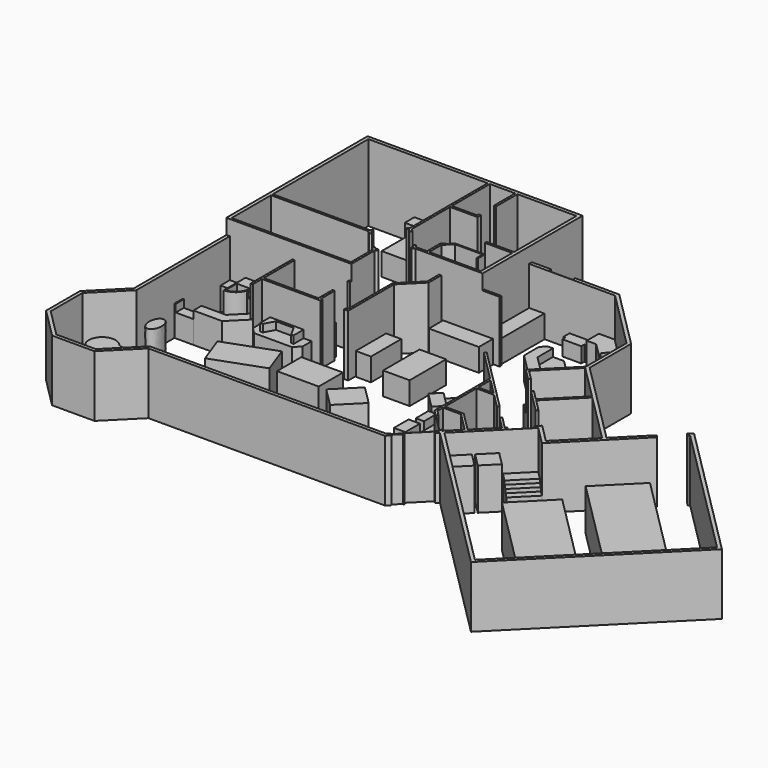
from build123d import *

# Parameters (mm, degrees)
F1_DEPTH  = 3076.575
F0_W      = 609.6
F0_H      = 1219.2
F2_DEPTH  = 914.4
F0_W_2    = 558.8
F0_H_2    = 482.6
F0_W_3    = 1676.4
F0_H_3    = 2438.4
F0_W_4    = 482.6
F0_H_4    = 1473.2
F0_W_5    = 355.6
F0_H_5    = 762
F0_W_6    = 457.2
F0_H_6    = 457.2
F3_DEPTH  = 609.6
F4_W      = 88.9
F4_H      = 76.2
F4_H_2    = 88.9
F5_DEPTH  = 2466.975
F6_DEPTH  = 1219.2
F4_W_2    = 1676.4
F4_H_3    = 1219.2
F4_W_3    = 889
F4_H_4    = 762
F4_W_4    = 1016
F4_H_5    = 381
F4_W_5    = 330.2
F4_H_6    = 635
F4_W_6    = 457.2
F4_H_7    = 736.6
F4_H_8    = 508
F4_W_7    = 1524
F4_H_9    = 457.2
F4_W_8    = 50.8
F4_H_10   = 406.4
F7_DEPTH  = 914.4
F4_W_9    = 622.3
F4_H_11   = 469.9
F4_W_10   = 711.2
F8_W      = 685.8
F8_H      = 88.9
F8_W_2    = 76.2
F8_W_3    = 965.2
F8_H_2    = 6.35
F9_DEPTH  = 2466.975
F8_W_4    = 609.6
F8_H_3    = 1524
F10_DEPTH = 914.4
F8_W_5    = 1066.8
F8_H_4    = 1828.8
F8_W_6    = 2006.6
F8_H_5    = 711.2
F8_R      = 114.3
F11_DEPTH = 609.6
F13_DEPTH = 2466.975
F14_DEPTH = 914.4
F12_W     = 685.8
F12_H     = 355.6
F15_DEPTH = 762
F16_DEPTH = 609.6
F18_DEPTH = 2466.975
F19_DEPTH = 1676.4


# Not quite as in the source:
# - a feature names something its author has since deleted; it is built from what else it names


with BuildPart() as f1:
    # F0 (on Top) → F1 (new body)
    with BuildSketch(Plane.XY):
        Polygon((-1281.9462310372, 633.3950885865), (-1281.9462310372, 1090.5950885865), (-824.7462310372, 1090.5950885865), (94.7987193947, 1090.5950885865), (1090.5950885865, 1090.5950885865), (1090.5950885865, 94.7987193947), (1090.5950885865, -824.7462310372), (1090.5950885865, -2043.9462310372), (480.9950885865, -2043.9462310372), (-14.3049114135, -2043.9462310372), (-14.3049114135, -2132.8462310372), (1090.5950885865, -2132.8462310372), (1090.5950885865, -3707.6462310372), (-986.9836923831, -3707.6462310372), (-986.9836923831, -3098.0462310372), (-682.1836923831, -2793.2462310372), (430.1950885865, -2793.2462310372), (430.1950885865, -3098.0462310372), (480.9950885865, -3098.0462310372), (480.9950885865, -2742.4462310372), (-703.2257413517, -2742.4462310372), (-915.1416434146, -2954.3621331001), (-942.0824117778, -2927.4213647369), (-1075.8836923831, -3061.2226453422), (-1075.8836923831, -3707.6462310372), (-1506.7811311724, -3707.6462310372), (-1614.5442046253, -3599.8831575844), (-1677.4059974727, -3662.7449504319), (-1569.6429240199, -3770.5080238847), (-1623.5244607463, -3824.3895606111), (-1560.6626678988, -3887.2513534586), (-1469.9575454775, -3796.5462310372), (1230.2950885865, -3796.5462310372), (1230.2950885865, 152.6643540582), (1230.2950885865, 1230.2950885865), (152.6643540582, 1230.2950885865), (-6336.0568161326, 1230.2950885865), (-7413.6875506609, 1230.2950885865), (-7413.6875506609, 152.6643540582), (-7413.6875506609, -5866.6462310372), (-2386.8462310372, -5866.6462310372), (-2386.8462310372, -4713.4349165969), (-2296.1411086158, -4622.7297941756), (-2359.0029014633, -4559.8680013281), (-2412.8844381897, -4613.7495380545), (-2520.6475116425, -4505.9864646017), (-2583.50930449, -4568.8482574492), (-2475.7462310372, -4676.611330902), (-2475.7462310372, -5777.7462310372), (-7273.9875506609, -5777.7462310372), (-7273.9875506609, -3796.5462310372), (-3355.811330902, -3796.5462310372), (-3248.0482574491, -3904.30930449), (-3185.1864646017, -3841.4475116425), (-3292.9495380545, -3733.6844381897), (-3239.0680013281, -3679.8029014633), (-3301.9297941756, -3616.9411086158), (-3392.6349165969, -3707.6462310372), (-6918.3875506609, -3707.6462310372), (-7273.9875506609, -3707.6462310372), (-7273.9875506609, -2945.6462310372), (-7273.9875506609, -2640.8462310372), (-7273.9875506609, -1167.6462310372), (-7273.9875506609, 94.7987193946), (-7273.9875506609, 1090.5950885865), (-6278.1911814691, 1090.5950885865), (-5422.1462310372, 1090.5950885865), (-4863.3462310372, 1090.5950885865), (-4787.1462310372, 1090.5950885865), (-3110.7462310372, 1090.5950885865), (-3034.5462310372, 1090.5950885865), (-2475.7462310372, 1090.5950885865), (-2475.7462310372, 607.9950885865), (-2475.7462310372, -2790.7575454775), (-2566.4513534586, -2881.4626678988), (-2503.5895606111, -2944.3244607463), (-2449.7080238847, -2890.4429240199), (-2341.9449504319, -2998.2059974727), (-2279.0831575844, -2935.3442046253), (-2386.8462310372, -2827.5811311724), (-2386.8462310372, -2585.9072780781), (-2386.8462310372, -909.5072780781), (-1777.2462310372, -909.5072780781), (-1281.9462310372, -909.5072780781), (-1281.9462310372, -820.6072780781), (-1281.9462310372, -744.4072780781), (-1370.8462310372, -744.4072780781), (-1370.8462310372, -820.6072780781), (-2386.8462310372, -820.6072780781), (-2386.8462310372, 1090.5950885865), (-1370.8462310372, 1090.5950885865), (-1370.8462310372, 17.5927219219), (-1281.9462310372, 17.5927219219), align=None)
    extrude(amount=F1_DEPTH)

    # F4 (on Top) → F5 (join)
    with BuildSketch(Plane.XY):
        Polygon((-7273.9875506609, -5866.6462310372), (-7413.6875506609, -5866.6462310372), (-7413.6875506609, -10507.7805963737), (-8618.8845674344, -11712.9776131472), (-8618.8845674344, -13417.3835796), (-7413.6875506609, -14622.5805963736), (-5709.281584208, -14622.5805963736), (-4504.0845674344, -13417.3835796), (5003.0722012166, -13417.3835796), (5151.7524573376, -13268.703323479), (5120.3215609139, -13237.2724270553), (5371.7687323038, -12985.8252556653), (5403.1996287275, -13017.2561520891), (5439.1206532118, -12981.3351276048), (5358.2983481222, -12900.5128225152), (6040.7978133234, -12218.0133573139), (6121.6201184131, -12298.8356624035), (6858.0011203407, -11562.4546604759), (5991.0966946136, -10695.5502347487), (5229.0966946136, -10695.5502347487), (5229.0966946136, -8271.0625060034), (3959.293014693, -7001.2588260828), (3896.4312218455, -7064.1206189303), (5140.1966946136, -8307.8860916984), (5140.1966946136, -11101.8860916984), (6130.6003745341, -12092.2897716189), (6022.8373010813, -12200.0528450718), (6036.3076852629, -12213.5232292534), (5353.8082200616, -12896.0226944546), (5340.33783588, -12882.552310273), (5304.4168113958, -12918.4733347573), (5335.8477078195, -12949.9042311811), (5084.4005364296, -13201.351402571), (5052.9696400058, -13169.9205061472), (4945.206566553, -13277.6835796001), (-4561.950202098, -13277.6835796), (-5767.1472188716, -14482.8805963736), (-7355.8219159973, -14482.8805963736), (-8479.1845674344, -13359.5179449365), (-8479.1845674344, -11770.8432478107), (-7273.9875506609, -10565.6462310372), (-7273.9875506609, -8648.3200841315), (-7273.9875506609, -8241.9200841315), (-7273.9875506609, -6336.5462310372), align=None)
        Polygon((6696.3565101615, -11526.5336359916), (6193.4621673816, -12029.4279787715), (6139.5806306552, -11975.5464420451), (6081.2089658682, -12033.918106832), (5398.709500667, -11351.4186416307), (5457.0811654539, -11293.0469768438), (5229.0966946136, -11065.0625060034), (5229.0966946136, -10784.4502347487), (5954.2731089186, -10784.4502347487), align=None, mode=Mode.SUBTRACT)
        Polygon((-4759.3875506609, -6901.5734475404), (-4759.3875506609, -7476.3098392888), (-4759.3875506609, -7873.2462310372), (-4670.4875506609, -7873.2462310372), (-4670.4875506609, -7504.9462310372), (-4345.0193547867, -7504.9462310372), (-2998.8193547867, -7504.9462310372), (-2673.3511589125, -7504.9462310372), (-2386.8462310372, -7504.9462310372), (-2386.8462310372, -6704.8462310372), (-2475.7462310372, -6704.8462310372), (-2475.7462310372, -7416.0462310372), (-4670.4875506609, -7416.0462310372), (-4670.4875506609, -5866.6462310372), (-4759.3875506609, -5866.6462310372), (-4759.3875506609, -6336.5462310372), align=None)
        with Locations((-2431.2962310372, -5904.7462310372)):
            Rectangle(F4_W, F4_H)
        with Locations((-4714.9375506609, -7917.6962310372)):
            Rectangle(F4_W, F4_H_2)
    extrude(amount=F5_DEPTH)

    # F8 (on Top) → F9 (join)
    with BuildSketch(Plane.XY):
        with Locations((1573.1950885865, -3752.0962310372)):
            Rectangle(F8_W, F8_H)
        Polygon((2004.9950885865, -1321.5416434146), (1230.2950885865, -1321.5416434146), (1230.2950885865, -1461.2416434146), (2004.9950885865, -1461.2416434146), (2004.9950885865, -1454.8916434146), align=None)
        Polygon((2970.1950885865, -1321.5416434146), (2970.1950885865, -1454.8916434146), (2970.1950885865, -1461.2416434146), (4683.6642412751, -1461.2416434146), (6987.9344635613, -3765.5118657007), (6987.9344635613, -5805.0420654303), (5647.8073852128, -7145.1691437788), (5710.6691780603, -7208.0309366262), (7127.6344635613, -5791.0656511253), (7127.6344635613, -3707.6462310372), (4741.5298759387, -1321.5416434146), align=None)
        Polygon((-1370.8462310372, -7416.0462310372), (-1370.8462310372, -7504.9462310372), (-1205.7462310372, -7504.9462310372), (-1205.7462310372, -5202.6625551158), (-431.6390822039, -4428.5554062825), (-431.6390822039, -3796.5462310372), (-520.5390822039, -3796.5462310372), (-520.5390822039, -4391.7318205875), (-1294.6462310372, -5165.8389694208), (-1294.6462310372, -7416.0462310372), align=None)
        with Locations((-2348.7462310372, -7460.4962310372)):
            Rectangle(F8_W_2, F8_H)
        with Locations((2487.5950885865, -1458.0666434146)):
            Rectangle(F8_W_3, F8_H_2)
    extrude(amount=F9_DEPTH)

    # F12 (on Top) → F13 (join)
    with BuildSketch(Plane.XY):
        Polygon((7028.8516462295, -5889.848468457), (8396.7700366499, -7257.7668588774), (7141.4493613282, -8513.0875341992), (6798.7398987186, -8170.3780715896), (6744.8583619922, -8116.4965348632), (6681.9965691447, -8179.3583277107), (7626.3831918659, -9123.7449504319), (7689.2449847134, -9060.8831575844), (7635.363447987, -9007.001620858), (7204.3111541757, -8575.9493270466), (8459.6318294974, -7320.6286517249), (8890.6841233087, -7751.6809455362), (10417.3276638905, -9278.324486118), (9162.0069885687, -10533.6451614397), (8425.6259866411, -9797.2641595121), (8362.7641937936, -9860.1259523595), (8255.0011203407, -9967.8890258124), (8349.293809612, -10062.1817150836), (7738.6363933793, -10672.8391313163), (7644.343704108, -10578.5464420451), (7590.4621673816, -10632.4279787715), (7105.5283368439, -10147.4941482337), (7042.6665439964, -10210.3559410812), (7527.6003745341, -10695.289771619), (6759.218303009, -11463.6718431441), (6858.0011203407, -11562.4546604759), (7635.363447987, -10785.0923328297), (7689.2449847134, -10731.2107961033), (8425.6259866411, -9994.8297941756), (8757.8954631206, -10327.0992706551), (8959.9512258447, -10529.1550333792), (9162.0069885687, -10731.2107961033), (10614.893298554, -9278.324486118), (7127.6344635613, -5791.0656511253), align=None)
        Polygon((6116.2404335173, -7487.8786063883), (5773.5309709078, -7145.1691437788), (5710.6691780603, -7208.0309366262), (6107.2601773963, -7604.6219359622), (6170.1219702438, -7541.7601431147), align=None)
        Polygon((5229.0966946136, -8271.0625060034), (5229.0966946136, -8396.7860916984), (5851.3966946135, -9019.0860916984), (5229.0966946136, -9019.0860916984), (5229.0966946136, -9107.9860916984), (5940.2966946136, -9107.9860916984), (6503.8511767323, -9671.5405738171), (6566.7129695797, -9608.6787809696), align=None)
    extrude(amount=F13_DEPTH)

    # F17 (on Top) → F18 (join)
    with BuildSketch(Plane.XY):
        Polygon((6328.1660091977, -12092.289771619), (6229.3831918659, -12191.0725889507), (12470.6611960089, -18432.3505930938), (18074.3410155561, -12828.6707735467), (12470.661196009, -7224.9909539995), (12317.9968419508, -7377.6553080577), (12416.7796592826, -7476.4381253894), (12470.661196009, -7422.556588663), (17876.7753808926, -12828.6707735467), (12470.6611960089, -18234.7849584303), align=None)
        Polygon((10516.1104812222, -9179.5416687862), (10614.893298554, -9278.324486118), (11734.2801940813, -8158.9375905907), (11635.4973767496, -8060.1547732589), align=None)
    extrude(amount=F18_DEPTH)


with BuildPart() as f2:
    # F0 (on Top) → F2 (new body)
    with BuildSketch(Plane.XY):
        with Locations((785.7950885865, -1434.3462310372)):
            Rectangle(F0_W, F0_H)
        with BuildLine():
            add(Edge.make_bspline(
                [(734.9950885865, -1180.3462310372), (383.0423644885, -1180.3462310372), (559.0187265375, -1561.3462310372), (734.9950885865, -1942.3462310372), (910.9714506355, -1561.3462310372), (1086.9478126845, -1180.3462310372), (734.9950885865, -1180.3462310372)],
                knots=[0, 0, 0, 2.0943951024, 2.0943951024, 4.1887902048, 4.1887902048, 6.2831853072, 6.2831853072, 6.2831853072], degree=2, weights=[1, 0.5, 1, 0.5, 1, 0.5, 1]))
        make_face(mode=Mode.SUBTRACT)
    extrude(amount=F2_DEPTH)


with BuildPart() as f2b:
    # F0 (on Top) → F2, piece 2 (new body)
    with BuildSketch(Plane.XY):
        Polygon((-1777.2462310372, -2433.5072780781), (-1777.2462310372, -909.5072780781), (-2386.8462310372, -909.5072780781), (-2386.8462310372, -2585.9072780781), (-1929.6462310372, -2585.9072780781), align=None)
        with BuildLine():
            add(Edge.make_bspline(
                [(-2031.2462310372, -1925.5072780781), (-1679.2935069392, -1925.5072780781), (-1855.2698689882, -1544.5072780781), (-2031.2462310372, -1163.5072780781), (-2207.2225930862, -1544.5072780781), (-2383.1989551352, -1925.5072780781), (-2031.2462310372, -1925.5072780781)],
                knots=[0, 0, 0, 2.0943951024, 2.0943951024, 4.1887902048, 4.1887902048, 6.2831853072, 6.2831853072, 6.2831853072], degree=2, weights=[1, 0.5, 1, 0.5, 1, 0.5, 1]))
        make_face(mode=Mode.SUBTRACT)
    extrude(amount=F2_DEPTH)


with BuildPart() as f2c:
    # F0 (on Top) → F2, piece 3 (new body)
    with BuildSketch(Plane.XY):
        with Locations((-5142.7462310372, 849.2950885865)):
            Rectangle(F0_W_2, F0_H_2)
    extrude(amount=F2_DEPTH)


with BuildPart() as f2d:
    # F0 (on Top) → F2, piece 4 (new body)
    with BuildSketch(Plane.XY):
        with Locations((-3948.9462310372, -128.6049114135)):
            Rectangle(F0_W_3, F0_H_3)
    extrude(amount=F2_DEPTH)


with BuildPart() as f2e:
    # F0 (on Top) → F2, piece 5 (new body)
    with BuildSketch(Plane.XY):
        with Locations((-2755.1462310372, 849.2950885865)):
            Rectangle(F0_W_2, F0_H_2)
    extrude(amount=F2_DEPTH)


with BuildPart() as f2f:
    # F0 (on Top) → F2, piece 6 (new body)
    with BuildSketch(Plane.XY):
        with Locations((-7032.6875506609, -1904.2462310372)):
            Rectangle(F0_W_4, F0_H_4)
    extrude(amount=F2_DEPTH)


with BuildPart() as f2g:
    # F0 (on Top) → F2, piece 7 (new body)
    with BuildSketch(Plane.XY):
        with Locations((-7096.1875506609, -3326.6462310372)):
            Rectangle(F0_W_5, F0_H_5)
    extrude(amount=F2_DEPTH)


with BuildPart() as f2h:
    # F0 (on Top) → F2, piece 8 (new body)
    with BuildSketch(Plane.XY):
        with Locations((-1053.3462310372, 861.9950885865)):
            Rectangle(F0_W_6, F0_H_6)
    extrude(amount=F2_DEPTH)


with BuildPart() as f3:
    # F0 (on Top) → F3 (new body)
    with BuildSketch(Plane.XY):
        Polygon((94.7987193947, 1090.5950885865), (-824.7462310372, 1090.5950885865), (-824.7462310372, 633.3950885865), (-824.7462310372, -37.3583565854), (-37.3583565854, -824.7462310372), (480.9950885865, -824.7462310372), (1090.5950885865, -824.7462310372), (1090.5950885865, 94.7987193947), (1090.5950885865, 1090.5950885865), align=None)
        with BuildLine():
            add(Edge.make_bspline(
                [(646.578440717, -646.578440717), (1299.8573551173, 6.7004736833), (3.3502368416, 649.9286775586), (-1293.156881434, 1293.156881434), (-649.9286775586, -3.3502368416), (-6.7004736833, -1299.8573551173), (646.578440717, -646.578440717)],
                knots=[0, 0, 0, 2.0943951024, 2.0943951024, 4.1887902048, 4.1887902048, 6.2831853072, 6.2831853072, 6.2831853072], degree=2, weights=[1, 0.5, 1, 0.5, 1, 0.5, 1]))
        make_face(mode=Mode.SUBTRACT)
    extrude(amount=F3_DEPTH)


with BuildPart() as f6:
    # F4 (on Top) → F6 (new body)
    with BuildSketch(Plane.XY):
        Polygon((-2609.6755261771, -9084.0103363379), (-4614.6037018859, -9813.7445141375), (-4197.6127431432, -10959.4177573997), (-2192.6845674344, -10229.6835796), align=None)
    extrude(amount=F6_DEPTH)


with BuildPart() as f6b:
    # F4 (on Top) → F6, piece 2 (new body)
    with BuildSketch(Plane.XY):
        with Locations((-1049.6845674344, -9620.0835796)):
            Rectangle(F4_W_2, F4_H_3)
    extrude(amount=F6_DEPTH)


with BuildPart() as f6c:
    # F4 (on Top) → F6, piece 3 (new body)
    with BuildSketch(Plane.XY):
        Polygon((1709.761534358, -10121.9205061472), (955.4200201882, -9367.5789919774), (93.3154325656, -10229.6835796), (847.6569467354, -10984.0250937698), align=None)
    extrude(amount=F6_DEPTH)


with BuildPart() as f6d:
    # F4 (on Top) → F6, piece 4 (new body)
    with BuildSketch(Plane.XY):
        with Locations((-4200.5875506609, -7009.6462310372)):
            Rectangle(F4_W_3, F4_H_4)
    extrude(amount=F6_DEPTH)


with BuildPart() as f6e:
    # F4 (on Top) → F6, piece 5 (new body)
    with BuildSketch(Plane.XY):
        Polygon((-2501.1462310372, -6501.6462310372), (-3567.9462310372, -6501.6462310372), (-3567.9462310372, -6527.0462310372), (-3567.9462310372, -7390.6462310372), (-2501.1462310372, -7390.6462310372), (-2501.1462310372, -6527.0462310372), align=None)
        with Locations((-3034.5462310372, -6717.5462310372)):
            Rectangle(F4_W_4, F4_H_5, mode=Mode.SUBTRACT)
    extrude(amount=F6_DEPTH)


with BuildPart() as f6f:
    # F4 (on Top) → F6, piece 6 (new body)
    with BuildSketch(Plane.XY):
        Polygon((3115.8551804438, -8115.5168262267), (2774.6054478431, -8456.7665588273), (3403.223376318, -9085.3844873021), (3744.4731089186, -8744.1347547015), align=None)
    extrude(amount=F6_DEPTH)


with BuildPart() as f6g:
    # F4 (on Top) → F6, piece 7 (new body)
    with BuildSketch(Plane.XY):
        with Locations((3679.6966946136, -9692.1860916984)):
            Rectangle(F4_W_5, F4_H_6)
    extrude(amount=F6_DEPTH)


with BuildPart() as f6h:
    # F4 (on Top) → F6, piece 8 (new body)
    with BuildSketch(Plane.XY):
        with Locations((3616.1966946136, -10581.1860916984)):
            Rectangle(F4_W_6, F4_H_7)
    extrude(amount=F6_DEPTH)


with BuildPart() as f6i:
    # F4 (on Top) → F6, piece 9 (new body)
    with BuildSketch(Plane.XY):
        with Locations((4132.406566553, -12998.2835796)):
            Rectangle(F4_W_4, F4_H_8)
    extrude(amount=F6_DEPTH)


with BuildPart() as f6j:
    # F4 (on Top) → F6, piece 10 (new body)
    with BuildSketch(Plane.XY):
        with BuildLine():
            ThreePointArc((3281.506566553, -13252.2835796), (3472.006566553, -13061.7835796), (3281.506566553, -12871.2835796))
            Line((3281.506566553, -12871.2835796001), (2684.606566553, -12871.2835796001))
            Line((2684.606566553, -12871.2835796), (2684.606566553, -13252.2835796))
            Line((2684.606566553, -13252.2835796), (3281.506566553, -13252.2835796))
        make_face()
    extrude(amount=F6_DEPTH)


with BuildPart() as f6k:
    # F4 (on Top) → F6, piece 11 (new body)
    with BuildSketch(Plane.XY):
        with Locations((-3183.2845674344, -12845.8835796)):
            Rectangle(F4_W_4, F4_H_4)
    extrude(amount=F6_DEPTH)


with BuildPart() as f6l:
    # F4 (on Top) → F6, piece 12 (new body)
    with BuildSketch(Plane.XY):
        Polygon((-6225.7143451483, -13540.5277677636), (-5974.2671737583, -13791.9749391535), (-5435.4518064942, -13253.1595718893), (-5686.8989778841, -13001.7124004994), align=None)
    extrude(amount=F6_DEPTH)


with BuildPart() as f6m:
    # F4 (on Top) → F6, piece 13 (new body)
    with BuildSketch(Plane.XY):
        with BuildLine():
            Line((-7662.5553245194, -12642.5021556566), (-6746.5692001703, -13558.4882800057))
            Line((-6746.5692001703, -13558.4882800057), (-5668.938465642, -12480.8575454774))
            Line((-5668.938465642, -12480.8575454774), (-6099.9907594533, -12049.8052516661))
            ThreePointArc((-6099.9907594532, -12049.805251666), (-6289.8110096941, -11948.216536705), (-6504.1022849014, -11968.9829465764))
            ThreePointArc((-6504.1022849014, -11968.9829465764), (-6718.3935601087, -11989.7493564478), (-6908.2138103495, -11888.1606414868))
            ThreePointArc((-6908.2138103495, -11888.1606414868), (-7662.5553245193, -11888.1606414868), (-7662.5553245194, -12642.5021556566))
        make_face()
    extrude(amount=F6_DEPTH)


with BuildPart() as f6n:
    # F4 (on Top) → F6, piece 14 (new body)
    with BuildSketch(Plane.XY):
        with BuildLine():
            add(Edge.make_bspline(
                [(-6873.1369972229, -10508.4746231079), (-6433.1960921004, -10508.4746231079), (-6653.1665446617, -9898.8746231079), (-6873.1369972229, -9289.2746231079), (-7093.1074497841, -9898.8746231079), (-7313.0779023454, -10508.4746231079), (-6873.1369972229, -10508.4746231079)],
                knots=[0, 0, 0, 2.0943951024, 2.0943951024, 4.1887902048, 4.1887902048, 6.2831853072, 6.2831853072, 6.2831853072], degree=2, weights=[1, 0.5, 1, 0.5, 1, 0.5, 1]))
        make_face()
    extrude(amount=F6_DEPTH)


with BuildPart() as f6o:
    # F4 (on Top) → F6, piece 15 (new body)
    with BuildSketch(Plane.XY):
        with Locations((-1049.6845674344, -12998.2835796)):
            Rectangle(F4_W_7, F4_H_9)
    extrude(amount=F6_DEPTH)


with BuildPart() as f6p:
    # F4 (on Top) → F6, piece 16 (new body)
    with BuildSketch(Plane.XY):
        with BuildLine():
            Line((-5407.0875506609, -5892.0462310372), (-6626.2875506609, -5892.0462310372))
            Line((-6626.2875506609, -5892.0462310372), (-6626.2875506609, -6374.6462310372))
            Line((-6626.2875506609, -6374.6462310372), (-6626.2875506609, -6984.2462310372))
            ThreePointArc((-6626.2875506609, -6984.2462310372), (-6195.2352568496, -6805.6985248485), (-6016.6875506609, -6374.6462310372))
            ThreePointArc((-6016.6875506609, -6374.6462310372), (-5838.1398444722, -6805.6985248485), (-5407.0875506609, -6984.2462310372))
            Line((-5407.0875506609, -6984.2462310372), (-5407.0875506609, -6374.6462310372))
            Line((-5407.0875506609, -6374.6462310372), (-5407.0875506609, -5892.0462310372))
        make_face()
        with BuildLine():
            Line((-6588.1875506609, -6944.8748167815), (-6588.1875506609, -6374.6462310372))
            Line((-6588.1875506609, -6374.6462310372), (-6054.7875506609, -6374.6462310372))
            ThreePointArc((-6054.7875506609, -6374.6462310372), (-6208.9229618419, -6765.0550552203), (-6588.1875506609, -6944.8748167815))
        make_face(mode=Mode.SUBTRACT)
        with BuildLine():
            Line((-5978.5875506609, -6374.6462310372), (-5445.1875506609, -6374.6462310372))
            Line((-5445.1875506609, -6374.6462310372), (-5445.1875506609, -6944.8748167815))
            ThreePointArc((-5445.1875506609, -6944.8748167815), (-5824.4521394798, -6765.0550552203), (-5978.5875506609, -6374.6462310372))
        make_face(mode=Mode.SUBTRACT)
    extrude(amount=F6_DEPTH)


with BuildPart() as f6q:
    # F4 (on Top) → F6, piece 17 (new body)
    with BuildSketch(Plane.XY):
        Polygon((-6461.1875506609, -8241.9200841315), (-6511.9875506609, -8241.9200841315), (-6511.9875506609, -8648.3200841315), (-5356.6614037552, -8648.3200841315), (-5253.752917925, -8545.4115983013), (-4750.8585751452, -8042.5172555215), (-4670.4875506609, -7962.1462310372), (-4759.3875506609, -7962.1462310372), (-4759.3875506609, -7873.2462310372), (-4759.3875506609, -7476.3098392888), (-5524.9977955036, -8241.9200841315), align=None)
    extrude(amount=F6_DEPTH)


with BuildPart() as f6r:
    # F4 (on Top) → F6, piece 18 (new body)
    with BuildSketch(Plane.XY):
        with Locations((-7248.5875506609, -8445.1200841315)):
            Rectangle(F4_W_8, F4_H_10)
    extrude(amount=F6_DEPTH)


with BuildPart() as f6s:
    # F4 (on Top) → F6, piece 19 (new body)
    with BuildSketch(Plane.XY):
        Polygon((-2998.8193547867, -7504.9462310372), (-4345.0193547867, -7504.9462310372), (-4345.0193547867, -8000.2462310372), (-4243.4193547867, -8000.2462310372), (-4027.5193547867, -7606.5462310372), (-3316.3193547867, -7606.5462310372), (-3100.4193547867, -8000.2462310372), (-2998.8193547867, -8000.2462310372), align=None)
    extrude(amount=F6_DEPTH)


with BuildPart() as f7:
    # F4 (on Top) → F7 (new body)
    with BuildSketch(Plane.XY):
        Polygon((5140.1966946136, -8307.8860916984), (3896.4312218455, -7064.1206189303), (2998.4056097386, -7962.1462310372), (3870.1966946136, -8833.9373159122), (3870.1966946136, -11101.8860916984), (5140.1966946136, -11101.8860916984), align=None)
    extrude(amount=F7_DEPTH)


with BuildPart() as f7b:
    # F4 (on Top) → F7, piece 2 (new body)
    with BuildSketch(Plane.XY):
        with Locations((-5070.5375506609, -6101.5962310372)):
            Rectangle(F4_W_9, F4_H_11)
    extrude(amount=F7_DEPTH)


with BuildPart() as f7c:
    # F4 (on Top) → F7, piece 3 (new body)
    with BuildSketch(Plane.XY):
        with Locations((-6962.8375506609, -6101.5962310372)):
            Rectangle(F4_W_9, F4_H_11)
    extrude(amount=F7_DEPTH)


with BuildPart() as f7d:
    # F4 (on Top) → F7, piece 4 (new body)
    with BuildSketch(Plane.XY):
        Polygon((-6461.1875506609, -7835.5200841315), (-6461.1875506609, -8241.9200841315), (-5524.9977955036, -8241.9200841315), (-4759.3875506609, -7476.3098392888), (-4759.3875506609, -6901.5734475404), (-5693.3341872521, -7835.5200841315), align=None)
    extrude(amount=F7_DEPTH)


with BuildPart() as f7e:
    # F4 (on Top) → F7, piece 5 (new body)
    with BuildSketch(Plane.XY):
        with Locations((-6867.5875506609, -8445.1200841315)):
            Rectangle(F4_W_10, F4_H_10)
    extrude(amount=F7_DEPTH)


with BuildPart() as f7f:
    # F4 (on Top) → F7, piece 6 (new body)
    with BuildSketch(Plane.XY):
        Polygon((-4670.4875506609, -7873.2462310372), (-4670.4875506609, -7962.1462310372), (-4429.1875506609, -8203.4462310372), (-2914.6511589125, -8203.4462310372), (-2673.3511589125, -7962.1462310372), (-2673.3511589125, -7504.9462310372), (-2998.8193547867, -7504.9462310372), (-2998.8193547867, -8000.2462310372), (-3100.4193547867, -8000.2462310372), (-3316.3193547867, -7606.5462310372), (-4027.5193547867, -7606.5462310372), (-4243.4193547867, -8000.2462310372), (-4345.0193547867, -8000.2462310372), (-4345.0193547867, -7504.9462310372), (-4670.4875506609, -7504.9462310372), align=None)
    extrude(amount=F7_DEPTH)


with BuildPart() as f10:
    # F8 (on Top) → F10 (new body)
    with BuildSketch(Plane.XY):
        with Locations((-875.5462310372, -6394.2094688416)):
            Rectangle(F8_W_4, F8_H_3)
    extrude(amount=F10_DEPTH)


with BuildPart() as f10b:
    # F8 (on Top) → F10, piece 2 (new body)
    with BuildSketch(Plane.XY):
        with Locations((851.6537689628, -6742.9462310372)):
            Rectangle(F8_W_5, F8_H_4)
    extrude(amount=F10_DEPTH)


with BuildPart() as f10c:
    # F8 (on Top) → F10, piece 3 (new body)
    with BuildSketch(Plane.XY):
        with Locations((664.3387786865, -4177.5462310372)):
            Rectangle(F8_W_6, F8_H_5)
    extrude(amount=F10_DEPTH)


with BuildPart() as f10d:
    # F8 (on Top) → F10, piece 4 (new body)
    with BuildSketch(Plane.XY):
        Polygon((1242.9950885865, -1473.9416434146), (1242.9950885865, -3694.9462310372), (1852.5950885865, -3694.9462310372), (1852.5950885865, -2780.5462310372), (1852.5950885865, -1473.9416434146), align=None)
    extrude(amount=F10_DEPTH)


with BuildPart() as f10e:
    # F8 (on Top) → F10, piece 5 (new body)
    with BuildSketch(Plane.XY):
        Polygon((4678.403729033, -1473.9416434146), (4044.8991414104, -1473.9416434146), (4044.8991414104, -2083.5416434146), (4425.8991414104, -2083.5416434146), (6365.6344635613, -4023.2769655655), (6365.6344635613, -5547.2769655655), (5988.4637064764, -5924.4477226504), (5754.9770473286, -5690.9610635026), (5108.3986066116, -6337.5395042196), (5341.8852657594, -6571.0261633674), (5207.7748352804, -6705.1365938464), (5638.8271290917, -7136.1888876577), (6975.2344635613, -5799.7815531881), (6975.2344635613, -3770.7723779429), align=None)
        with Locations((6505.3344635613, -5128.1769655655)):
            Circle(F8_R, mode=Mode.SUBTRACT)
        with Locations((6784.7344635613, -5128.1769655655)):
            Circle(F8_R, mode=Mode.SUBTRACT)
        with Locations((6505.3344635613, -4785.2769655655)):
            Circle(F8_R, mode=Mode.SUBTRACT)
        with Locations((6784.7344635613, -4785.2769655655)):
            Circle(F8_R, mode=Mode.SUBTRACT)
        with Locations((6505.3344635613, -4442.3769655655)):
            Circle(F8_R, mode=Mode.SUBTRACT)
        with Locations((6784.7344635613, -4442.3769655655)):
            Circle(F8_R, mode=Mode.SUBTRACT)
        with BuildLine():
            ThreePointArc((5198.2011678223, -2173.3442046253), (5252.0827045487, -2151.0257413517), (5305.9642412751, -2173.3442046253))
            Line((5305.9642412751, -2173.3442046253), (5844.7796085393, -2712.1595718894))
            ThreePointArc((5844.7796085393, -2712.1595718894), (5867.0980718129, -2766.0411086158), (5844.7796085393, -2819.9226453422))
            Line((5844.7796085393, -2819.9226453422), (5593.3324371494, -3071.3698167322))
            ThreePointArc((5593.3324371494, -3071.3698167322), (5539.4509004229, -3093.6882800058), (5485.5693636965, -3071.3698167322))
            Line((5485.5693636965, -3071.3698167322), (4946.7539964324, -2532.554449468))
            ThreePointArc((4946.7539964324, -2532.554449468), (4924.4355331588, -2478.6729127416), (4946.7539964324, -2424.7913760152))
            Line((4946.7539964324, -2424.7913760152), (5198.2011678223, -2173.3442046253))
        make_face(mode=Mode.SUBTRACT)
    extrude(amount=F10_DEPTH)


with BuildPart() as f10f:
    # F8 (on Top) → F10, piece 6 (new body)
    with BuildSketch(Plane.XY):
        Polygon((3541.6950885865, -3150.3416434146), (3338.4950885865, -3150.3416434146), (3135.2950885865, -3353.5416434146), (3135.2950885865, -4097.6718431441), (4115.3740641022, -5077.7508186598), (4859.5042638317, -5077.7508186598), (5062.7042638317, -4874.5508186598), (5062.7042638317, -4671.3508186598), (4283.7104558506, -4671.3508186598), (3541.6950885865, -3929.3354513957), align=None)
    extrude(amount=F10_DEPTH)


with BuildPart() as f11:
    # F8 (on Top) → F11 (new body)
    with BuildSketch(Plane.XY):
        Polygon((3984.0161130707, -3150.3416434146), (3541.6950885865, -3150.3416434146), (3541.6950885865, -3929.3354513957), (4283.7104558506, -4671.3508186598), (5062.7042638317, -4671.3508186598), (5062.7042638317, -4229.0297941756), align=None)
    extrude(amount=F11_DEPTH)


with BuildPart() as f11b:
    # F8 (on Top) → F11, piece 2 (new body)
    with BuildSketch(Plane.XY):
        Polygon((3856.9526672363, -1569.8820688248), (2942.5526672363, -1569.8820688248), (2942.5526672363, -1874.6820688248), (3018.7526672363, -1874.6820688248), (3018.7526672363, -2027.0820688248), (3780.7526672363, -2027.0820688248), (3780.7526672363, -1874.6820688248), (3856.9526672363, -1874.6820688248), align=None)
    extrude(amount=F11_DEPTH)


with BuildPart() as f14:
    # F12 (on Top) → F14 (new body)
    with BuildSketch(Plane.XY):
        with BuildLine():
            add(Edge.make_bspline(
                [(5610.0966946136, -9361.9860916984), (5258.1439705156, -9361.9860916984), (5434.1203325646, -9762.0360916984), (5610.0966946136, -10162.0860916984), (5786.0730566626, -9762.0360916984), (5962.0494187116, -9361.9860916984), (5610.0966946136, -9361.9860916984)],
                knots=[0, 0, 0, 2.0943951024, 2.0943951024, 4.1887902048, 4.1887902048, 6.2831853072, 6.2831853072, 6.2831853072], degree=2, weights=[1, 0.5, 1, 0.5, 1, 0.5, 1]))
        make_face()
    extrude(amount=F14_DEPTH)


with BuildPart() as f14b:
    # F12 (on Top) → F14, piece 2 (new body)
    with BuildSketch(Plane.XY):
        Polygon((5864.0966946136, -9133.3860916984), (5356.0966946136, -9133.3860916984), (5356.0966946136, -9361.9860916984), (5610.0966946136, -9361.9860916984), (5864.0966946136, -9361.9860916984), align=None)
    extrude(amount=F14_DEPTH)


with BuildPart() as f14c:
    # F12 (on Top) → F14, piece 3 (new body)
    with BuildSketch(Plane.XY):
        with Locations((5597.3966946136, -10492.3502347487)):
            Rectangle(F12_W, F12_H)
    extrude(amount=F14_DEPTH)


with BuildPart() as f14d:
    # F12 (on Top) → F14, piece 4 (new body)
    with BuildSketch(Plane.XY):
        Polygon((6999.7252408344, -10396.9813421803), (6460.9098735703, -10935.7967094444), (6856.0411428973, -11330.9279787715), (7394.8565101615, -10792.1126115073), align=None)
        with BuildLine():
            add(Edge.make_bspline(
                [(7143.4093387716, -10648.4285135702), (6894.5411809048, -10399.5603557034), (6695.6860394797, -10847.2836549953), (6496.8308980546, -11295.0069542872), (6944.5541973464, -11096.1518128621), (7392.2774966383, -10897.296671437), (7143.4093387716, -10648.4285135702)],
                knots=[0, 0, 0, 2.0943951024, 2.0943951024, 4.1887902048, 4.1887902048, 6.2831853072, 6.2831853072, 6.2831853072], degree=2, weights=[1, 0.5, 1, 0.5, 1, 0.5, 1]))
        make_face(mode=Mode.SUBTRACT)
    extrude(amount=F14_DEPTH)


with BuildPart() as f14e:
    # F12 (on Top) → F14, piece 5 (new body)
    with BuildSketch(Plane.XY):
        Polygon((9815.6505037789, -8730.5288627328), (9276.8351365147, -9269.3442299969), (9815.6505037788, -9808.1595972611), (10354.465871043, -9269.3442299969), align=None)
    extrude(amount=F14_DEPTH)


with BuildPart() as f14f:
    # F12 (on Top) → F14, piece 6 (new body)
    with BuildSketch(Plane.XY):
        Polygon((9153.0267324477, -9393.152634064), (8614.2113651835, -9931.9680013281), (9153.0267324477, -10470.7833685923), (9691.8420997118, -9931.9680013281), align=None)
    extrude(amount=F14_DEPTH)


with BuildPart() as f14g:
    # F12 (on Top) → F14, piece 7 (new body)
    with BuildSketch(Plane.XY):
        Polygon((7204.3111541757, -8575.9493270466), (7635.363447987, -9007.001620858), (8890.6841233087, -7751.6809455362), (8459.6318294974, -7320.6286517249), align=None)
    extrude(amount=F14_DEPTH)


with BuildPart() as f14h:
    # F12 (on Top) → F14, piece 8 (new body)
    with BuildSketch(Plane.XY):
        Polygon((7141.4493613282, -8513.0875341992), (8396.7700366499, -7257.7668588774), (7028.8516462295, -5889.848468457), (5773.5309709078, -7145.1691437788), (6116.2404335173, -7487.8786063883), (6403.6086293916, -7200.5104105141), (6348.2673626562, -7145.1691437788), (7028.8516462295, -6464.5848602054), (7822.0336449015, -7257.7668588774), (7141.4493613282, -7938.3511424507), (7086.1080945928, -7883.0098757154), (6798.7398987186, -8170.3780715896), align=None)
    extrude(amount=F14_DEPTH)


with BuildPart() as f14i:
    # F12 (on Top) → F14, piece 9 (new body)
    with BuildSketch(Plane.XY):
        Polygon((7967.6329244665, -11117.3618093092), (8757.8954631206, -10327.0992706551), (8425.6259866411, -9994.8297941756), (7689.2449847134, -10731.2107961033), (7635.363447987, -10785.0923328297), align=None)
    extrude(amount=F14_DEPTH)


with BuildPart() as f15:
    # F12 (on Top) → F15 (new body)
    with BuildSketch(Plane.XY):
        Polygon((8169.6886871906, -11319.4175720333), (8959.9512258447, -10529.1550333792), (8757.8954631206, -10327.0992706551), (7967.6329244665, -11117.3618093092), align=None)
    extrude(amount=F15_DEPTH)


with BuildPart() as f16:
    # F12 (on Top) → F16 (new body)
    with BuildSketch(Plane.XY):
        Polygon((8371.7444499146, -11521.4733347573), (9162.0069885687, -10731.2107961033), (8959.9512258447, -10529.1550333792), (8169.6886871906, -11319.4175720333), align=None)
    extrude(amount=F16_DEPTH)


with BuildPart() as f19:
    # F17 (on Top) → F19 (new body)
    with BuildSketch(Plane.XY):
        Polygon((14512.1727541987, -15546.6949595236), (11099.6754281924, -12134.1976335173), (9752.637010032, -13481.2360516777), (13165.1343360383, -16893.733377684), align=None)
    extrude(amount=F19_DEPTH)


with BuildPart() as f19b:
    # F17 (on Top) → F19, piece 2 (new body)
    with BuildSketch(Plane.XY):
        Polygon((16535.7238001463, -13523.143913576), (12548.4900823916, -9535.9101958213), (11111.6491030205, -10972.7511751924), (15098.8828207752, -14959.9848929471), align=None)
    extrude(amount=F19_DEPTH)


with BuildPart() as f19c:
    # F17 (on Top) → F19, piece 3 (new body)
    with BuildSketch(Plane.XY):
        Polygon((7585.4018661474, -10906.8959636378), (7046.5864988832, -11445.711330902), (7585.4018661473, -11984.5266981661), (8124.2172334115, -11445.711330902), align=None)
    extrude(amount=F19_DEPTH)


with BuildPart() as f19d:
    # F17 (on Top) → F19, piece 4 (new body)
    with BuildSketch(Plane.XY):
        Polygon((6974.7444499146, -11517.5533798705), (6435.9290826505, -12056.3687471347), (6974.7444499146, -12595.1841143988), (7513.5598171788, -12056.3687471347), align=None)
    extrude(amount=F19_DEPTH)


solid = Compound([f1.part, f2.part, f2b.part, f2c.part, f2d.part, f2e.part, f2f.part, f2g.part, f2h.part, f3.part, f6.part, f6b.part, f6c.part, f6d.part, f6e.part, f6f.part, f6g.part, f6h.part, f6i.part, f6j.part, f6k.part, f6l.part, f6m.part, f6n.part, f6o.part, f6p.part, f6q.part, f6r.part, f6s.part, f7.part, f7b.part, f7c.part, f7d.part, f7e.part, f7f.part, f10.part, f10b.part, f10c.part, f10d.part, f10e.part, f10f.part, f11.part, f11b.part, f14.part, f14b.part, f14c.part, f14d.part, f14e.part, f14f.part, f14g.part, f14h.part, f14i.part, f15.part, f16.part, f19.part, f19b.part, f19c.part, f19d.part])
